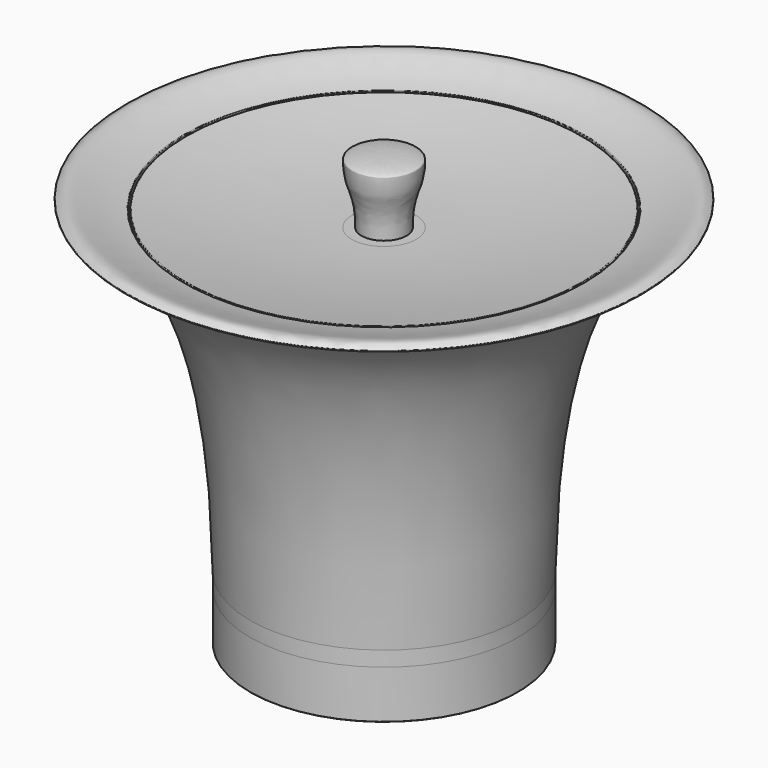
from build123d import *


# Not quite as in the source:
# - ends of sketch curves that miss each other by under 0.0002 mm in the source are joined


with BuildPart() as f1:
    # F0 (on Front) → F1 (revolve)
    with BuildSketch(Plane.XZ):
        with BuildLine():
            ThreePointArc((-39.2, -15), (-39.0585786438, -14.9414213562), (-39, -14.8))
            Line((-39, -14.8), (-39, -0.2))
            ThreePointArc((-39, -0.2), (-38.9414213562, -0.0585786438), (-38.8, 0))
            Line((-38.8, 0), (-34.3236067977, 0))
            ThreePointArc((-34.3236067977, 0), (-34.1534766361, 0.0948537776), (-34.1447213595, 0.2894427191))
            Line((-34.1447213596, 0.2894427191), (-36.88854382, 5.77708764))
            ThreePointArc((-36.88854382, 5.77708764), (-38.4649797894, 10.126301139), (-39, 14.72135955))
            Line((-39, 14.72135955), (-39, 29.1675041929))
            ThreePointArc((-39, 29.1675041929), (-44.1087470692, 63.8085203443), (-59, 95.5))
            Line((-59, 95.5), (-61.9414213562, 98.4414213562))
            ThreePointArc((-61.9414213562, 98.4414213562), (-61.9847759065, 98.506306026), (-62, 98.5828427125))
            Line((-62, 98.5828427125), (-62, 103.3308152157))
            ThreePointArc((-62, 103.3308152157), (-62.0472149133, 103.459876121), (-62.1665671727, 103.5280010318))
            add(Edge.make_bspline(
                [(-79.7040573299, 106.2801035961), (-76.3260555853, 109.2943212913), (-73.531506087, 105.4549248188), (-62.1665671727, 103.5280010318)],
                knots=[0.510348349, 0.510348349, 0.510348349, 0.510348349, 18.0872261708, 18.0872261708, 18.0872261708, 18.0872261708], degree=3))
            ThreePointArc((-79.7040573299, 106.2801035961), (-79.7632452463, 106.0760736715), (-79.6054125719, 105.9338756882))
            add(Edge.make_bspline(
                [(-79.6054125719, 105.9338756882), (-53.0177693175, 101.275930607), (-42.1177251641, 58.2548807339), (-41.5256360973, 4.6772239645)],
                knots=[0.5380548431, 0.5380548431, 0.5380548431, 0.5380548431, 109.6185883344, 109.6185883344, 109.6185883344, 109.6185883344], degree=3))
            add(Edge.make_bspline(
                [(-41.5256360973, 4.6772239645), (-41.5085019086, 3.1267651973), (-41.5, 1.5674659193), (-41.5, 0)],
                knots=[109.6185883344, 109.6185883344, 109.6185883344, 109.6185883344, 112.7752189091, 112.7752189091, 112.7752189091, 112.7752189091], degree=3))
            Line((-41.5, 0), (-41.5, -14.8))
            ThreePointArc((-41.5, -14.8), (-41.4414213562, -14.9414213562), (-41.3, -15))
            Line((-41.3, -15), (-39.2, -15))
        make_face()
    revolve(axis=Axis((0, 0, 53), (0, 0, 1)))


with BuildPart() as f3:
    # F2 (on Front) → F3 (revolve)
    with BuildSketch(Plane.XZ):
        with BuildLine():
            ThreePointArc((-61.5, 98.7899494937), (-61.4847759065, 98.7134128072), (-61.4414213562, 98.6485281374))
            Line((-61.4414213562, 98.6485281374), (-60.8917539568, 98.098860738))
            ThreePointArc((-60.8917539568, 98.098860738), (-60.825593446, 98.0696749898), (-60.7570536431, 98.0927252936))
            ThreePointArc((-60.7570536431, 98.0927252936), (-59.4100505063, 98.0313708499), (-59.3486960627, 96.6843677131))
            ThreePointArc((-59.3486960627, 96.6843677131), (-59.3717463664, 96.6158279103), (-59.3425606183, 96.5496673995))
            Line((-59.3425606183, 96.5496673995), (-58.7928932188, 96))
            ThreePointArc((-58.7928932188, 96), (-58.728008549, 95.9566454497), (-58.6514718626, 95.9414213562))
            Line((-58.6514718626, 95.9414213562), (-53.9946369043, 95.9414213562))
            ThreePointArc((-53.9946369043, 95.9414213562), (-53.8360391332, 96.0195741282), (-53.8013899164, 96.1929538863))
            Line((-53.8013899164, 96.1929538863), (-54.4568182455, 98.6508101206))
            ThreePointArc((-54.4568182455, 98.6508101206), (-54.4134872982, 98.8347253564), (-54.236347346, 98.9004811342))
            Line((-54.236347346, 98.9004811342), (-32.7, 95.9414213562))
            Line((-32.7, 95.9414213562), (-2.9, 95.9414213562))
            ThreePointArc((-2.9, 95.9414213562), (-2.7585786438, 96), (-2.7, 96.1414213562))
            Line((-2.7, 96.1414213562), (-2.7, 98.2414213562))
            ThreePointArc((-2.7, 98.2414213562), (-2.7585786438, 98.3828427125), (-2.9, 98.4414213562))
            Line((-2.9, 98.4414213562), (-10, 98.4414213562))
            add(Edge.make_bspline(
                [(-61.2671212492, 103.3778470888), (-49.4321558211, 101.4047526307), (-31.8561846668, 98.4414213562), (-10, 98.4414213562)],
                knots=[0.3382259655, 0.3382259655, 0.3382259655, 0.3382259655, 51.7397629092, 51.7397629092, 51.7397629092, 51.7397629092], degree=3))
            ThreePointArc((-61.2671212492, 103.3778470888), (-61.4292749792, 103.3331785788), (-61.5, 103.1805745823))
            Line((-61.5, 103.1805745823), (-61.5, 98.7899494937))
        make_face()
    revolve(axis=Axis((0, 0, 53), (0, 0, 1)))


with BuildPart() as f5:
    # F4 (on Front) → F5 (revolve)
    with BuildSketch(Plane.XZ):
        with BuildLine():
            Line((0, 98.4414213562), (0, 118.4414213562))
            add(Edge.make_bspline(
                [(0, 118.4414213562), (-6, 118.4414213562), (-10, 117.9414213562), (-10, 116.9414213562)],
                knots=[0, 0, 0, 0, 10.1118742081, 10.1118742081, 10.1118742081, 10.1118742081], degree=3))
            add(Edge.make_bspline(
                [(-10, 116.9414213562), (-10, 108.9414213562), (-7.0000002161, 109.4414213562), (-7.0000002161, 98.4414213562)],
                knots=[0, 0, 0, 0, 18.7416647794, 18.7416647794, 18.7416647794, 18.7416647794], degree=3))
            Line((-7.0000002161, 98.4414213562), (0, 98.4414213562))
        make_face()
    revolve(axis=Axis((0, 0, 108.4414213562), (0, 0, -1)))


solid = Compound([f1.part, f3.part, f5.part])
